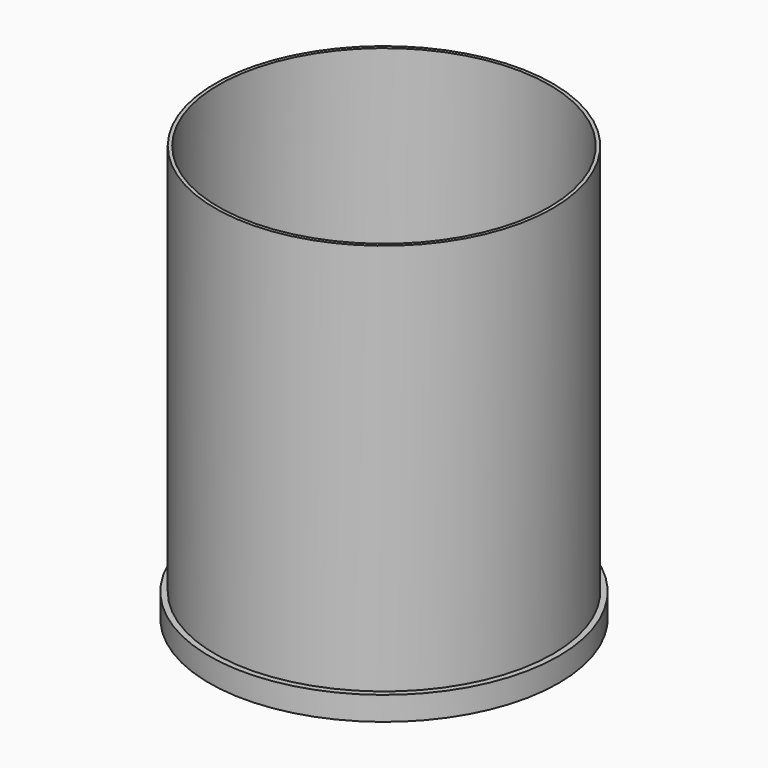
from build123d import *

# Parameters (mm, degrees)
F0_R      = 75
F1_DEPTH  = 5
F0_R_2    = 79
F2_DEPTH  = 30
F3_R      = 142.5
F3_R_2    = 79
F3_R_3    = 75
F4_DEPTH  = 5
F3_R_4    = 145.5
F5_DEPTH  = 158
F6_DEPTH  = 180
F7_R      = 150.5
F7_R_2    = 145.5
F7_R_3    = 142.5
F8_DEPTH  = 7.5
F9_R      = 150.5
F9_R_2    = 147
F10_DEPTH = 13
F11_R     = 6.5
F11_R_2   = 3.5
F12_DEPTH = 7
F13_D     = 6.6
F13_DEPTH = 12
F13_TIP   = 1.9828400428


with BuildPart() as f1:
    # F0 (on Top) → F1 (new body)
    with BuildSketch(Plane.XY):
        Circle(F0_R)
        with BuildLine():
            ThreePointArc((-27.2772727273, 3.4929060339), (0, 27.5), (27.2772727273, 3.4929060339))
            ThreePointArc((27.2772727273, 3.4929060339), (31, 0), (27.2772727273, -3.4929060339))
            ThreePointArc((27.2772727273, -3.4929060339), (0, -27.5), (-27.2772727273, -3.4929060339))
            ThreePointArc((-27.2772727273, -3.4929060339), (-31, 0), (-27.2772727273, 3.4929060339))
        make_face(mode=Mode.SUBTRACT)
    extrude(amount=F1_DEPTH)

    # F0 (on Top) → F2 (join)
    with BuildSketch(Plane.XY):
        Circle(F0_R_2)
        Circle(F0_R, mode=Mode.SUBTRACT)
    extrude(amount=F2_DEPTH)

    # F3 (on face) → F4 (join)
    with BuildSketch(Plane.XY.offset(30)):
        Circle(F3_R)
        Circle(F3_R_2, mode=Mode.SUBTRACT)
        Circle(F3_R_2)
        Circle(F3_R_3, mode=Mode.SUBTRACT)
    extrude(amount=F4_DEPTH)

    # F3 (on face) → F5 (join)
    with BuildSketch(Plane.XY.offset(30)):
        Circle(F3_R_4)
        Circle(F3_R, mode=Mode.SUBTRACT)
    extrude(amount=F5_DEPTH)

    # F3 (on face) → F6 (join)
    with BuildSketch(Plane.XY.offset(30)):
        Circle(F3_R_4)
        Circle(F3_R, mode=Mode.SUBTRACT)
    extrude(amount=-F6_DEPTH)

    # F7 (on face) → F8 (join)
    with BuildSketch(Plane(origin=(0, 0, -150), x_dir=(1, 0, 0), z_dir=(0, 0, -1))):
        Circle(F7_R)
        Circle(F7_R_2, mode=Mode.SUBTRACT)
        Circle(F7_R_2)
        Circle(F7_R_3, mode=Mode.SUBTRACT)
    extrude(amount=F8_DEPTH)

    # F9 (on face) → F10 (join)
    with BuildSketch(Plane(origin=(0, 0, -157.5), x_dir=(1, 0, 0), z_dir=(0, 0, -1))):
        Circle(F9_R)
        Circle(F9_R_2, mode=Mode.SUBTRACT)
    extrude(amount=F10_DEPTH)

    # F11 (on face) → F12 (join)
    with BuildSketch(Plane.XY.offset(35)):
        with Locations((0, 82.1006134727)):
            Circle(F11_R)
        with Locations((0, 82.1006134727)):
            Circle(F11_R_2, mode=Mode.SUBTRACT)
        with Locations((65.5, -49.5001084099)):
            Circle(F11_R)
        with Locations((65.5, -49.5001084099)):
            Circle(F11_R_2, mode=Mode.SUBTRACT)
        with Locations((-65.5, -49.5001084099)):
            Circle(F11_R)
        with Locations((-65.5, -49.5001084099)):
            Circle(F11_R_2, mode=Mode.SUBTRACT)
    extrude(amount=F12_DEPTH)

    # F13
    with Locations(Plane.XY.offset(35)):
        with Locations((0, 82.1006134727), (65.5, -49.5001084099), (-65.5, -49.5001084099)):
            Hole(F13_D / 2, depth=F13_DEPTH)
            with Locations((0, 0, -(F13_DEPTH + F13_TIP / 2))):  # 118° drill point
                Cone(0, F13_D / 2, F13_TIP, mode=Mode.SUBTRACT)


solid = f1.part
